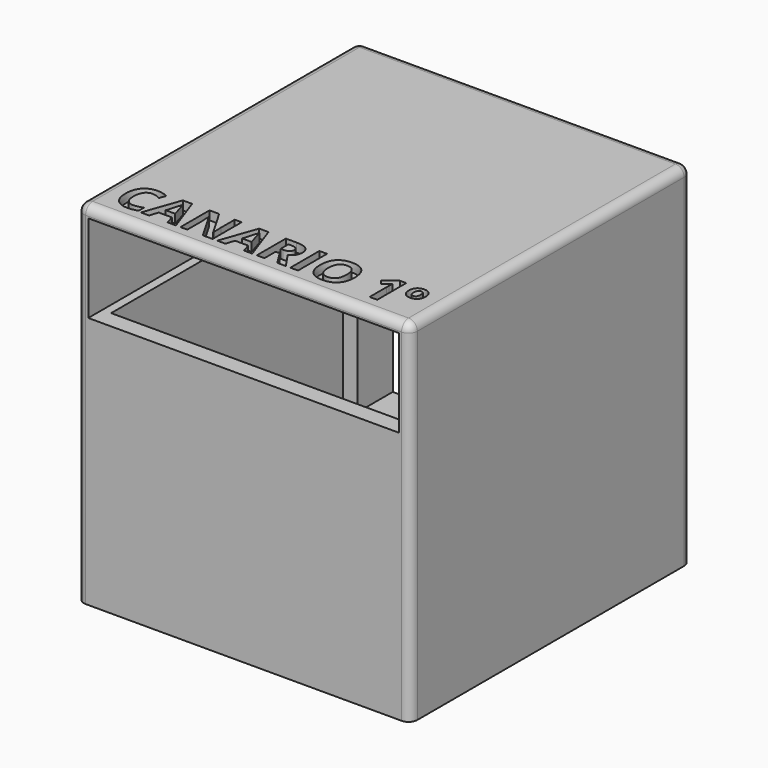
from build123d import *

# Parameters (mm, degrees)
F0_W          = 190
F0_H          = 200
F1_DEPTH      = 200
F2_W          = 177
F2_H          = 50
F3_DEPTH      = 190
F4_W          = 167
F4_H          = 165
F5_DEPTH      = 120
F6_W          = 60
F6_H          = 30
F6_W_2        = 50
F7_DEPTH      = 10.001
F9_DEPTH      = 25
F10_W         = 150
F10_H         = 141
F11_DEPTH     = 5
F12_W         = 140
F12_H         = 131
F13_DEPTH     = 19.001
F14_W         = 140
F14_H         = 14
F15_DEPTH     = 30.001
F16_R         = 2
F17_DEPTH     = 10.001
F18_TEXT_SIZE = 28.9477185047
F19_DEPTH     = 5
F20_R         = 5


# Not quite as in the source:
# - Text() gives the source's letters only with a copy of the font that has no kerning and outlines rounded to 1/6400 em; it was checked with that copy


with BuildPart() as f1:
    # F0 (on Top) → F1 (new body)
    with BuildSketch(Plane.XY):
        with Locations((95, -100)):
            Rectangle(F0_W, F0_H)
    extrude(amount=F1_DEPTH)

    # F2 (on face) → F3 (cut)
    with BuildSketch(Plane.XZ.offset(200)):
        with Locations((95, 169)):
            Rectangle(F2_W, F2_H)
    extrude(amount=-F3_DEPTH, mode=Mode.SUBTRACT)

    # F4 (on face) → F5 (cut)
    with BuildSketch(Plane.XY.offset(144)):
        with Locations((95, -107.5)):
            Rectangle(F4_W, F4_H)
    extrude(amount=-F5_DEPTH, mode=Mode.SUBTRACT)

    # F6 (on face) → F7 (cut, through all)
    with BuildSketch(Plane.XZ.offset(10)):
        with Locations((36.5, 159)):
            Rectangle(F6_W, F6_H)
        with Locations((158.5, 159)):
            Rectangle(F6_W_2, F6_H)
    extrude(amount=-F7_DEPTH, mode=Mode.SUBTRACT)

    # F8 (on face) → F9 (cut, through all)
    with BuildSketch(Plane(origin=(0, 0, 0), x_dir=(-1, 0, 0), z_dir=(0, 1, 0))):
        Polygon((-170, 125), (-170, 30), (-95, 30), (-20, 30), (-20, 125), align=None)
    extrude(amount=-F9_DEPTH, mode=Mode.SUBTRACT)

    # F10 (on face) → F11 (cut)
    with BuildSketch(Plane.XY.offset(24)):
        with Locations((95, -95.5)):
            Rectangle(F10_W, F10_H)
    extrude(amount=-F11_DEPTH, mode=Mode.SUBTRACT)

    # F12 (on face) → F13 (cut, through all)
    with BuildSketch(Plane.XY.offset(19)):
        with Locations((95, -95.5)):
            Rectangle(F12_W, F12_H)
    extrude(amount=-F13_DEPTH, mode=Mode.SUBTRACT)

    # F14 (on face) → F15 (cut, through all)
    with BuildSketch(Plane.XZ.offset(30)):
        with Locations((95, 7)):
            Rectangle(F14_W, F14_H)
    extrude(amount=-F15_DEPTH, mode=Mode.SUBTRACT)

    # F16 (on face) → F17 (cut, through all)
    with BuildSketch(Plane.XZ.offset(10)):
        with Locations((93.5, 169)):
            Circle(F16_R)
    extrude(amount=-F17_DEPTH, mode=Mode.SUBTRACT)

    # F18 (on face) → F19 (cut)
    with BuildSketch(Plane.XY.offset(200)):
        with Locations((10, -190)):
            Text('CANARIO 1º', F18_TEXT_SIZE, font='Open Sans', font_style=FontStyle.BOLD, text_align=(TextAlign.LEFT, TextAlign.BOTTOM))
    extrude(amount=-F19_DEPTH, mode=Mode.SUBTRACT)

    # F20
    f20_edges = [f1.edges().sort_by_distance(p)[0] for p in [
        (190, -100, 200),
        (95, -200, 200),
        (190, -200, 100),
        (0, -100, 200),
        (0, -200, 100),
        (0, 0, 100),
        (95, 0, 200),
        (190, 0, 100),
    ]]
    fillet(f20_edges, radius=F20_R)


solid = f1.part
